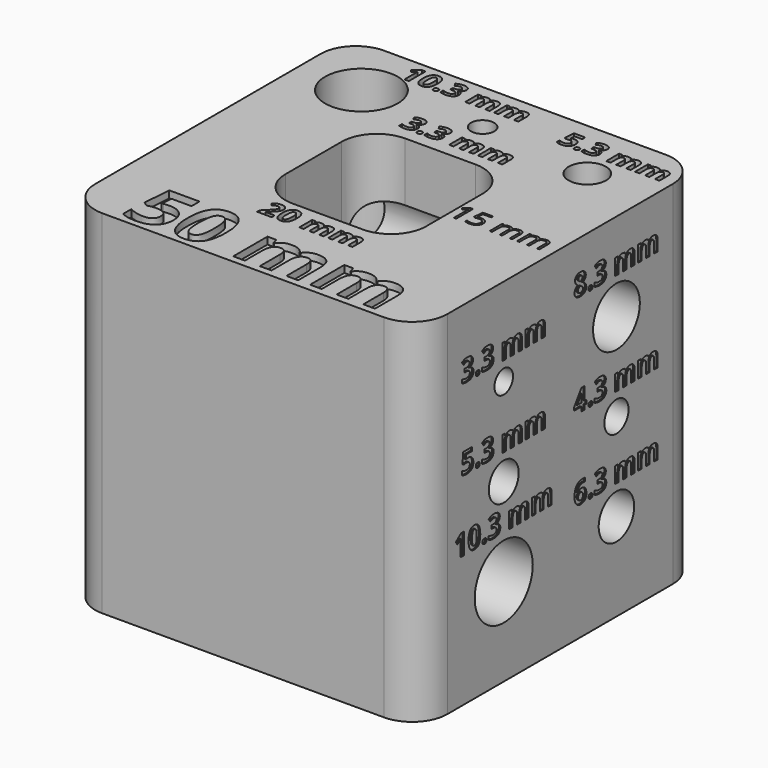
from build123d import *

# Parameters (mm, degrees)
F0_W            = 50
F0_H            = 50
F1_DEPTH        = 50
F2_W            = 20
F2_H            = 20
F3_DEPTH        = 50.001
F4_R            = 5
F5_R            = 5
F6_R            = 5.15
F6_R_2          = 1.65
F6_R_3          = 2.65
F7_DEPTH        = 50.001
F8_R            = 1.65
F8_R_2          = 2.65
F8_R_3          = 5.15
F8_R_4          = 4.15
F8_R_5          = 2.15
F8_R_6          = 3.15
F9_DEPTH        = 50.001
F10_TEXT_SIZE   = 4.1666666667
F11_DEPTH       = 0.2
F12_TEXT_SIZE   = 11.1111111111
F12_TEXT_SIZE_2 = 4.1666666667
F13_DEPTH       = 1


# Not quite as in the source:
# - Text() gives the source's letters only with a copy of the font that has no kerning and outlines rounded to 1/6400 em; it was checked with that copy


with BuildPart() as f1:
    # F0 (on Top) → F1 (new body)
    with BuildSketch(Plane.XY):
        Rectangle(F0_W, F0_H)
    extrude(amount=F1_DEPTH)

    # F2 (on face) → F3 (cut, through all)
    with BuildSketch(Plane.XY.offset(50)):
        Rectangle(F2_W, F2_H)
    extrude(amount=-F3_DEPTH, mode=Mode.SUBTRACT)

    # F4
    f4_edges = [f1.edges().sort_by_distance(p)[0] for p in [
        (-25, 25, 25),
        (25, 25, 25),
        (25, -25, 25),
        (-25, -25, 25),
    ]]
    fillet(f4_edges, radius=F4_R)

    # F5
    f5_edges = [f1.edges().sort_by_distance(p)[0] for p in [
        (10, 10, 25),
        (-10, 10, 25),
        (10, -10, 25),
        (-10, -10, 25),
    ]]
    fillet(f5_edges, radius=F5_R)

    # F6 (on face) → F7 (cut, through all)
    with BuildSketch(Plane.XY.offset(50)):
        with Locations((-16.0355339059, 16.0355339059)):
            Circle(F6_R)
        with Locations((0, 17.5)):
            Circle(F6_R_2)
        with Locations((16.0355339059, 16.0355339059)):
            Circle(F6_R_3)
    extrude(amount=-F7_DEPTH, mode=Mode.SUBTRACT)

    # F8 (on face) → F9 (cut, through all)
    with BuildSketch(Plane.YZ.offset(25)):
        with Locations((-10, 37.5)):
            Circle(F8_R)
        with Locations((-10, 25)):
            Circle(F8_R_2)
        with Locations((-10, 12.5)):
            Circle(F8_R_3)
        with Locations((10, 37.5)):
            Circle(F8_R_4)
        with Locations((10, 25)):
            Circle(F8_R_5)
        with Locations((10, 12.5)):
            Circle(F8_R_6)
    extrude(amount=-F9_DEPTH, mode=Mode.SUBTRACT)

    # F10 (on face) → F11 (cut)
    with BuildSketch(Plane.YZ.offset(25)):
        with Locations((-17.5843098958, 28.65)):
            Text('5.3 mm', F10_TEXT_SIZE, font='Open Sans', font_style=FontStyle.BOLD, text_align=(TextAlign.LEFT, TextAlign.BOTTOM))
        with Locations((-18.7734375, 18.65)):
            Text('10.3 mm', F10_TEXT_SIZE, font='Open Sans', font_style=FontStyle.BOLD, text_align=(TextAlign.LEFT, TextAlign.BOTTOM))
        with Locations((-17.5843098958, 40.15)):
            Text('3.3 mm', F10_TEXT_SIZE, font='Open Sans', font_style=FontStyle.BOLD, text_align=(TextAlign.LEFT, TextAlign.BOTTOM))
        with Locations((2.4156901042, 42.65)):
            Text('8.3 mm', F10_TEXT_SIZE, font='Open Sans', font_style=FontStyle.BOLD, text_align=(TextAlign.LEFT, TextAlign.BOTTOM))
        with Locations((2.4156901042, 28.15)):
            Text('4.3 mm', F10_TEXT_SIZE, font='Open Sans', font_style=FontStyle.BOLD, text_align=(TextAlign.LEFT, TextAlign.BOTTOM))
        with Locations((2.4156901042, 16.65)):
            Text('6.3 mm', F10_TEXT_SIZE, font='Open Sans', font_style=FontStyle.BOLD, text_align=(TextAlign.LEFT, TextAlign.BOTTOM))
    extrude(amount=-F11_DEPTH, mode=Mode.SUBTRACT)

    # F12 (on face) → F13 (cut)
    with BuildSketch(Plane.XY.offset(50)):
        with Locations((-18.640625, -24)):
            Text('50 mm', F12_TEXT_SIZE, font='Open Sans', font_style=FontStyle.BOLD, text_align=(TextAlign.LEFT, TextAlign.BOTTOM))
        with Locations((10, -1.5)):
            Text('15 mm', F12_TEXT_SIZE_2, font='Open Sans', text_align=(TextAlign.LEFT, TextAlign.BOTTOM))
        with Locations((-7.5843098958, 11.85)):
            Text('3.3 mm', F12_TEXT_SIZE_2, font='Open Sans', font_style=FontStyle.BOLD, text_align=(TextAlign.LEFT, TextAlign.BOTTOM))
        with Locations((-15, 21)):
            Text('10.3 mm', F12_TEXT_SIZE_2, font='Open Sans', font_style=FontStyle.BOLD, text_align=(TextAlign.LEFT, TextAlign.BOTTOM))
        with Locations((8.4512240101, 19.6855339059)):
            Text('5.3 mm', F12_TEXT_SIZE_2, font='Open Sans', font_style=FontStyle.BOLD, text_align=(TextAlign.LEFT, TextAlign.BOTTOM))
        with Locations((-6.990234375, -14)):
            Text('20 mm', F12_TEXT_SIZE_2, font='Open Sans', font_style=FontStyle.BOLD, text_align=(TextAlign.LEFT, TextAlign.BOTTOM))
    extrude(amount=-F13_DEPTH, mode=Mode.SUBTRACT)


solid = f1.part
